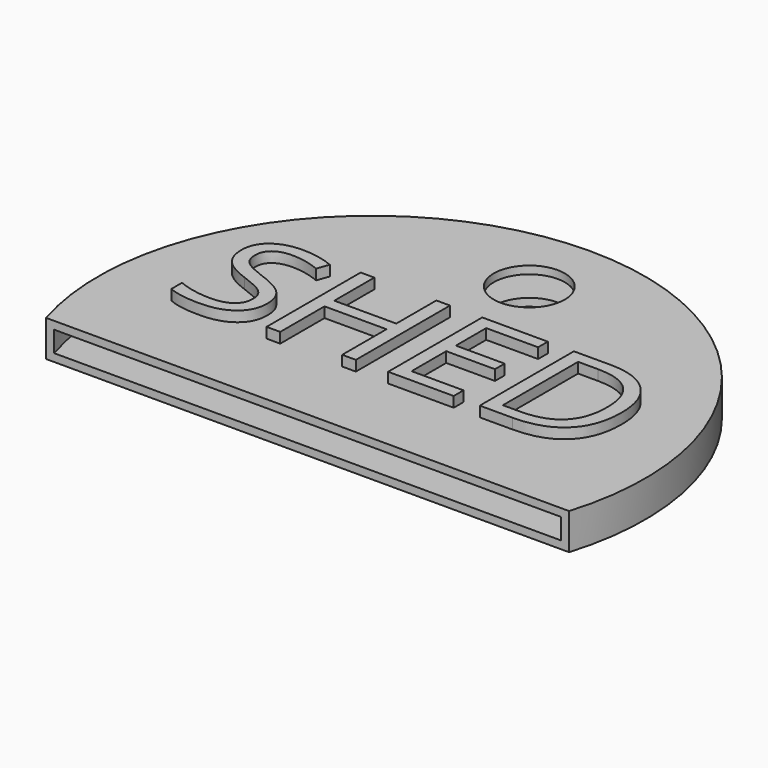
from build123d import *

# Parameters (mm, degrees)
F1_DEPTH     = 3.5
F2_T         = -1.5
F3_R         = 6.8535823447
F4_DEPTH     = 7.001
F5_TEXT_SIZE = 31.8145896826
F6_DEPTH     = 2


# Not quite as in the source:
# - Text() gives the source's letters only with a copy of the font that has no kerning and outlines rounded to 1/6400 em; it was checked with that copy


with BuildPart() as f1:
    # F0 (on Top) → F1 (new body, symmetric)
    with BuildSketch(Plane.XY):
        with BuildLine():
            Line((-50.4859743441, -15.4682988907), (50.4859743441, -15.4682988907))
            ThreePointArc((50.4859743441, -15.4682988907), (0, 52.8024798285), (-50.4859743441, -15.4682988907))
        make_face()
    extrude(amount=F1_DEPTH, both=True)

    # F2
    f2_openings = [f1.faces().sort_by_distance(p)[0] for p in [
        (0, -15.468299, 0),
    ]]
    offset(amount=F2_T, openings=f2_openings)

    # F3 (on face) → F4 (cut, through all)
    with BuildSketch(Plane.XY.offset(3.5)):
        with Locations((0, 38.0384922028)):
            Circle(F3_R)
    extrude(amount=-F4_DEPTH, mode=Mode.SUBTRACT)

    # F5 (on face) → F6 (join)
    with BuildSketch(Plane.XY.offset(3.5)):
        with Locations((-40.881183671, 0)):
            Text('SHED', F5_TEXT_SIZE, font='Open Sans', text_align=(TextAlign.LEFT, TextAlign.BOTTOM))
    extrude(amount=F6_DEPTH)


solid = f1.part
